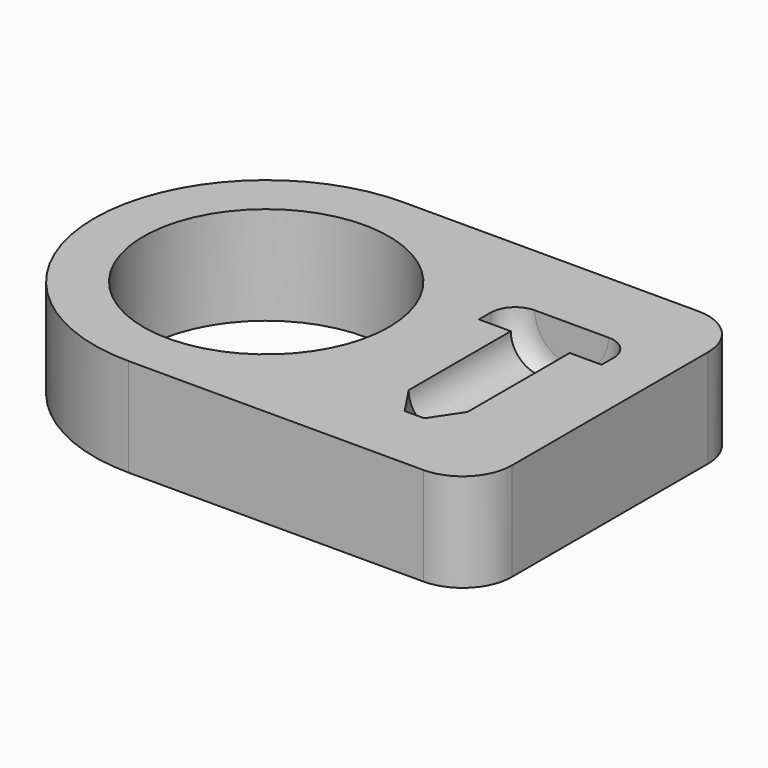
from build123d import *

# Parameters (mm, degrees)
F0_R         = 12.5
F1_DEPTH     = 10
F4_TEXT_SIZE = 5.5555555556
F5_DEPTH     = 1


# Not quite as in the source:
# - Text() gives the source's letters only with a copy of the font that has no kerning and outlines rounded to 1/6400 em; it was checked with that copy


with BuildPart() as f1:
    # F0 (on Top) → F1 (new body)
    with BuildSketch(Plane.XY):
        with BuildLine():
            ThreePointArc((0, 17.5), (5.1256313292, 5.1256313292), (17.5, 0))
            Line((17.5, 0), (47.5, 0))
            ThreePointArc((47.5, 0), (51.0355339059, 1.4644660941), (52.5, 5))
            Line((52.5, 5), (52.5, 30))
            ThreePointArc((52.5, 30), (51.0355339059, 33.5355339059), (47.5, 35))
            Line((47.5, 35), (17.5, 35))
            ThreePointArc((17.5, 35), (5.1256313292, 29.8743686708), (0, 17.5))
        make_face()
        with Locations((17.5, 17.5)):
            Circle(F0_R, mode=Mode.SUBTRACT)
    extrude(amount=F1_DEPTH)

    # F2 (on face) → F3 (revolve, cut)
    with BuildSketch(Plane.XY.offset(10)):
        with BuildLine():
            Line((41, 23), (41, 7))
            Line((41, 7), (42, 7))
            Line((42, 7), (44, 10))
            Line((44, 10), (44, 23))
            Line((44, 23), (47.25, 23))
            Line((47.25, 23), (47.25, 24.5))
            ThreePointArc((47.25, 24.5), (46.517766953, 26.267766953), (44.75, 27))
            Line((44.75, 27), (41, 27))
            Line((41, 27), (41, 23))
        make_face()
    revolve(axis=Axis((41, 15, 10), (0, 1, 0)), mode=Mode.SUBTRACT)

    # F4 (on face) → F5 (cut)
    with BuildSketch(Plane(origin=(0, 0, 0), x_dir=(1, 0, 0), z_dir=(0, 0, -1))):
        with Locations((29, -9)):
            Text('904, 905', F4_TEXT_SIZE, font='Open Sans', text_align=(TextAlign.LEFT, TextAlign.BOTTOM))
    extrude(amount=-F5_DEPTH, mode=Mode.SUBTRACT)


solid = f1.part
